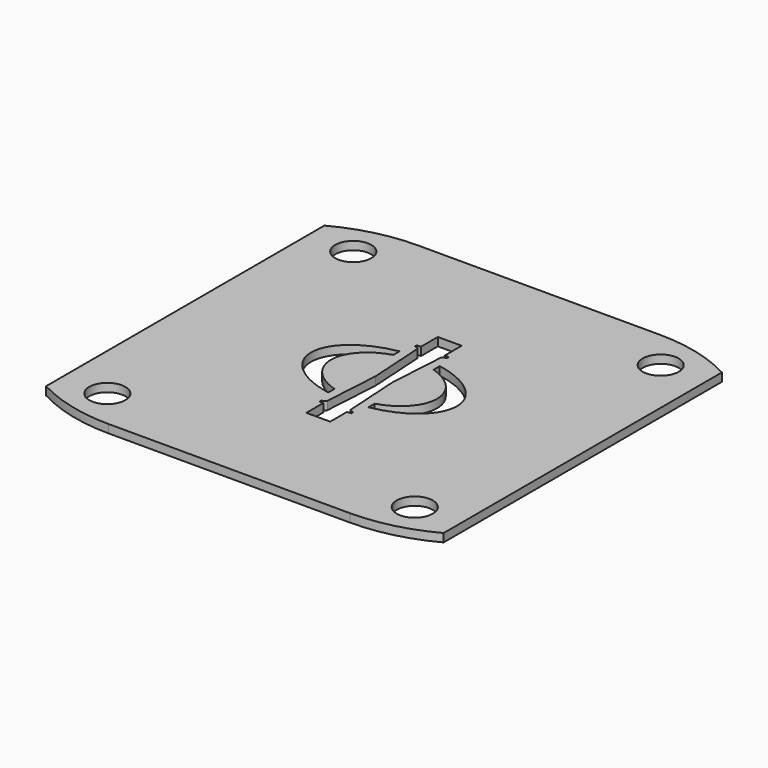
from build123d import *

# Parameters (mm, degrees)
F0_R     = 1.7272
F1_DEPTH = 0.79375
F3_DEPTH = 25.4


# Not quite as in the source:
# - a feature names something its author has since deleted; it is built from what else it names


with BuildPart() as f1:
    # F0 (on Top) → F1 (new body)
    with BuildSketch(Plane.XY):
        with BuildLine():
            Line((-19.05, 16.66875), (-19.05, 0))
            Line((-19.05, 0), (-19.05, -16.66875))
            ThreePointArc((-19.05, -16.66875), (-15.4310103444, -18.0612265152), (-11.5824, -18.5348037427))
            Line((-11.5824, -18.5348037427), (0, -18.5348037427))
            Line((0, -18.5348037427), (11.5824, -18.5348037427))
            ThreePointArc((11.5824, -18.5348037427), (15.4310103444, -18.0612265152), (19.05, -16.66875))
            Line((19.05, -16.66875), (19.05, 0))
            Line((19.05, 0), (19.05, 16.66875))
            ThreePointArc((19.05, 16.66875), (15.4310103444, 18.0612265152), (11.5824, 18.5348037427))
            Line((11.5824, 18.5348037427), (0, 18.5348037427))
            Line((0, 18.5348037427), (-11.5824, 18.5348037427))
            ThreePointArc((-11.5824, 18.5348037427), (-15.4310103444, 18.0612265152), (-19.05, 16.66875))
        make_face()
        with Locations((-14.732, -14.732)):
            Circle(F0_R, mode=Mode.SUBTRACT)
        with Locations((14.732, -14.732)):
            Circle(F0_R, mode=Mode.SUBTRACT)
        with Locations((-14.732, 14.732)):
            Circle(F0_R, mode=Mode.SUBTRACT)
        with Locations((14.732, 14.732)):
            Circle(F0_R, mode=Mode.SUBTRACT)
    extrude(amount=F1_DEPTH)

    # F2 (on face) → F3 (cut)
    with BuildSketch(Plane.XY.offset(0.79375)):
        with BuildLine():
            Line((-1.381887138, -5.588), (-1.524, -5.588))
            Line((-1.524, -5.588), (-1.524, -5.842))
            Line((-1.524, -5.842), (-1.143, -5.842))
            Line((-1.143, -5.842), (-1.143, -7.874))
            Line((-1.143, -7.874), (0, -7.874))
            Line((0, -7.874), (1.143, -7.874))
            Line((1.143, -7.874), (1.143, -5.842))
            Line((1.143, -5.842), (1.524, -5.842))
            Line((1.524, -5.842), (1.524, -5.588))
            Line((1.524, -5.588), (1.381887138, -5.588))
            ThreePointArc((1.381887138, -5.588), (1.2078708338, -5.5190252033), (1.128364287, -5.349561621))
            Line((1.128364287, -5.349561621), (0.8, 0))
            Line((0.8, 0), (1.128364287, 5.349561621))
            ThreePointArc((1.128364287, 5.349561621), (1.2078708338, 5.5190252033), (1.381887138, 5.588))
            Line((1.381887138, 5.588), (1.524, 5.588))
            Line((1.524, 5.588), (1.524, 5.842))
            Line((1.524, 5.842), (1.143, 5.842))
            Line((1.143, 5.842), (1.143, 7.874))
            Line((1.143, 7.874), (0, 7.874))
            Line((0, 7.874), (-1.143, 7.874))
            Line((-1.143, 7.874), (-1.143, 5.842))
            Line((-1.143, 5.842), (-1.524, 5.842))
            Line((-1.524, 5.842), (-1.524, 5.588))
            Line((-1.524, 5.588), (-1.381887138, 5.588))
            ThreePointArc((-1.381887138, 5.588), (-1.2078708338, 5.5190252033), (-1.128364287, 5.349561621))
            Line((-1.128364287, 5.349561621), (-0.8, 0))
            Line((-0.8, 0), (-1.128364287, -5.349561621))
            ThreePointArc((-1.128364287, -5.349561621), (-1.2078708338, -5.5190252033), (-1.381887138, -5.588))
        make_face()
        with BuildLine():
            add(Edge.make_bspline(
                [(-1.922114287, 3.5267450469), (-13.4260486871, 0), (-1.922114287, -3.5267450469)],
                knots=[1.958829942, 1.958829942, 1.958829942, 4.3243553652, 4.3243553652, 4.3243553652], degree=2, weights=[1, 0.3783689541, 1]))
            Line((-1.922114287, 3.5267450469), (-1.922114287, 4.2733939342))
            add(Edge.make_bspline(
                [(-1.922114287, 4.2733939342), (-25.3836232991, 0), (-1.922114287, -4.2733939342)],
                knots=[1.8495705702, 1.8495705702, 1.8495705702, 4.433614737, 4.433614737, 4.433614737], degree=2, weights=[1, 0.2751774212, 1]))
            Line((-1.922114287, -4.2733939342), (-1.922114287, -3.5267450469))
        make_face()
        with BuildLine():
            Line((1.922114287, 4.2733939342), (1.922114287, 3.5267450469))
            add(Edge.make_bspline(
                [(1.922114287, -3.5267450469), (13.4260486871, 0), (1.922114287, 3.5267450469)],
                knots=[5.1004225956, 5.1004225956, 5.1004225956, 7.4659480188, 7.4659480188, 7.4659480188], degree=2, weights=[1, 0.3783689541, 1]))
            Line((1.922114287, -3.5267450469), (1.922114287, -4.2733939342))
            add(Edge.make_bspline(
                [(1.922114287, -4.2733939342), (25.3836232991, 0), (1.922114287, 4.2733939342)],
                knots=[4.9911632238, 4.9911632238, 4.9911632238, 7.5752073906, 7.5752073906, 7.5752073906], degree=2, weights=[1, 0.2751774212, 1]))
        make_face()
    extrude(amount=-F3_DEPTH, mode=Mode.SUBTRACT)


solid = f1.part
